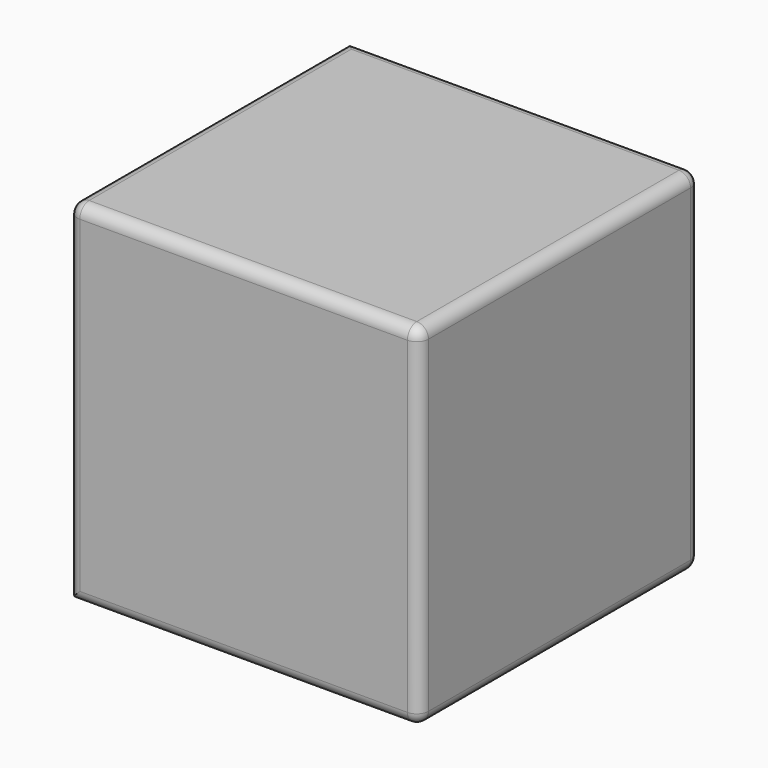
from build123d import *

# Parameters (mm, degrees)
F0_W         = 152.4
F0_H         = 152.4
F1_DEPTH     = 152.4
F2_R         = 5.08
F3_R         = 5.08
F4_R         = 5.08
F6_T1_DEPTH  = 154.94
F6_T3_DEPTH  = 142.24
F6_T5_DEPTH  = 142.24
F6_S9_W      = 5.1816
F6_S9_H      = 5.1816
F6_T10_DEPTH = 5.1816
F6_T14_ANGLE = 90
F6_T16_ANGLE = 90


# Not quite as in the source:
# - a fillet or chamfer that OpenCascade refuses, or shapes differently, is made with other operations: its cross-section is extruded or revolved along the edge and cut away or added
# - a feature of the source that left no trace in its solid (it failed there, or was rolled back) is left out


with BuildPart() as f1:
    # F0 (on Top) → F1 (new body)
    with BuildSketch(Plane.XY):
        with Locations((-37.6290231943, 42.0823047486)):
            Rectangle(F0_W, F0_H)
    extrude(amount=-F1_DEPTH)

    # F2
    f2_edges = [f1.edges().sort_by_distance(p)[0] for p in [
        (38.570977, -34.117695, -76.2),
    ]]
    fillet(f2_edges, radius=F2_R)

    # F3
    f3_edges = [f1.edges().sort_by_distance(p)[0] for p in [
        (38.570977, 44.622305, 0),
    ]]
    fillet(f3_edges, radius=F3_R)

    # F4
    f4_edges = [f1.edges().sort_by_distance(p)[0] for p in [
        (-113.829023, -34.117695, -78.74),
        (-113.829023, -32.629798, -1.487898),
        (-113.829023, 42.082305, -152.4),
        (-113.829023, 44.622305, 0),
        (-113.829023, 118.282305, -76.2),
    ]]
    fillet(f4_edges, radius=F4_R)

    # F6: fillet of radius 5.08 on 8 edges, made by hand

    # F6_s2 → F6_t1 (cut)
    with BuildSketch(Plane.YZ.offset(-121.4490231943)):
        with BuildLine():
            ThreePointArc((113.2023047486, -152.4), (116.794407197, -150.9121024484), (118.2823047486, -147.32))
            Line((118.2823047486, -147.32), (118.2823047486, -152.4))
            Line((118.2823047486, -152.4), (113.2023047486, -152.4))
        make_face()
        with BuildLine():
            ThreePointArc((113.2023047486, 0), (116.794407197, -1.4878975516), (118.2823047486, -5.08))
            Line((118.2823047486, -5.08), (118.2823047486, 0))
            Line((118.2823047486, 0), (113.2023047486, 0))
        make_face()
        with BuildLine():
            ThreePointArc((-34.1176952514, -147.32), (-32.6297976998, -150.9121024484), (-29.0376952514, -152.4))
            Line((-29.0376952514, -152.4), (-34.1176952514, -152.4))
            Line((-34.1176952514, -152.4), (-34.1176952514, -147.32))
        make_face()
    extrude(amount=F6_T1_DEPTH, mode=Mode.SUBTRACT)

    # F6_s4 → F6_t3 (cut)
    with BuildSketch(Plane.XY.offset(-147.32)):
        with BuildLine():
            ThreePointArc((38.5709768057, 113.2023047486), (37.0830792541, 116.794407197), (33.4909768057, 118.2823047486))
            Line((33.4909768057, 118.2823047486), (38.5709768057, 118.2823047486))
            Line((38.5709768057, 118.2823047486), (38.5709768057, 113.2023047486))
        make_face()
    extrude(amount=F6_T3_DEPTH, mode=Mode.SUBTRACT)

    # F6_s6 → F6_t5 (cut)
    with BuildSketch(Plane.XZ.offset(-113.2023047486)):
        with BuildLine():
            ThreePointArc((33.4909768057, -152.4), (37.0830792541, -150.9121024484), (38.5709768057, -147.32))
            Line((38.5709768057, -147.32), (38.5709768057, -152.4))
            Line((38.5709768057, -152.4), (33.4909768057, -152.4))
        make_face()
    extrude(amount=F6_T5_DEPTH, mode=Mode.SUBTRACT)


with BuildPart() as f6_tool8:
    # F6_s9 → F6_t10 (new body)
    with BuildSketch(Plane.YZ.offset(33.4909768057)):
        with Locations((115.7931047486, -149.9108)):
            Rectangle(F6_S9_W, F6_S9_H)
    extrude(amount=F6_T10_DEPTH)

    # F6_s11 → F6_t12 (revolve, cut)
    with BuildSketch(Plane(origin=(33.4909768057, 113.2023047486, -147.32), x_dir=(0, -0.7071067812, 0.7071067812), z_dir=(0, 0.7071067812, 0.7071067812))):
        with BuildLine():
            ThreePointArc((0, -5.08), (5.08, 0), (0, 5.08))
            Line((0, 5.08), (0, -5.08))
        make_face()
    revolve(axis=Axis((33.4909768057, 113.2023047486, -147.32), (1, 0, 0)), mode=Mode.SUBTRACT)


with BuildPart() as f1_1:
    add(f1.part)

    # F6_t7: cut F6_tool8
    add(f6_tool8.part, mode=Mode.SUBTRACT)

    # F6_s13 → F6_t14 (revolve, cut)
    with BuildSketch(Plane.YZ.offset(33.4909768057)):
        with BuildLine():
            ThreePointArc((118.2823047486, -5.08), (116.794407197, -1.4878975516), (113.2023047486, 0))
            Line((113.2023047486, 0), (118.2823047486, 0))
            Line((118.2823047486, 0), (118.2823047486, -5.08))
        make_face()
    revolve(axis=Axis((33.4909768057, 118.2823047486, -5.08), (0, 1, 0)), revolution_arc=F6_T14_ANGLE, mode=Mode.SUBTRACT)

    # F6_s15 → F6_t16 (revolve, cut)
    with BuildSketch(Plane.YZ.offset(33.4909768057)):
        with BuildLine():
            ThreePointArc((-34.1176952514, -147.32), (-32.6297976998, -150.9121024484), (-29.0376952514, -152.4))
            Line((-29.0376952514, -152.4), (-34.1176952514, -152.4))
            Line((-34.1176952514, -152.4), (-34.1176952514, -147.32))
        make_face()
    revolve(axis=Axis((33.4909768057, -29.0376952514, -152.4), (0, 0, 1)), revolution_arc=F6_T16_ANGLE, mode=Mode.SUBTRACT)


solid = f1_1.part
